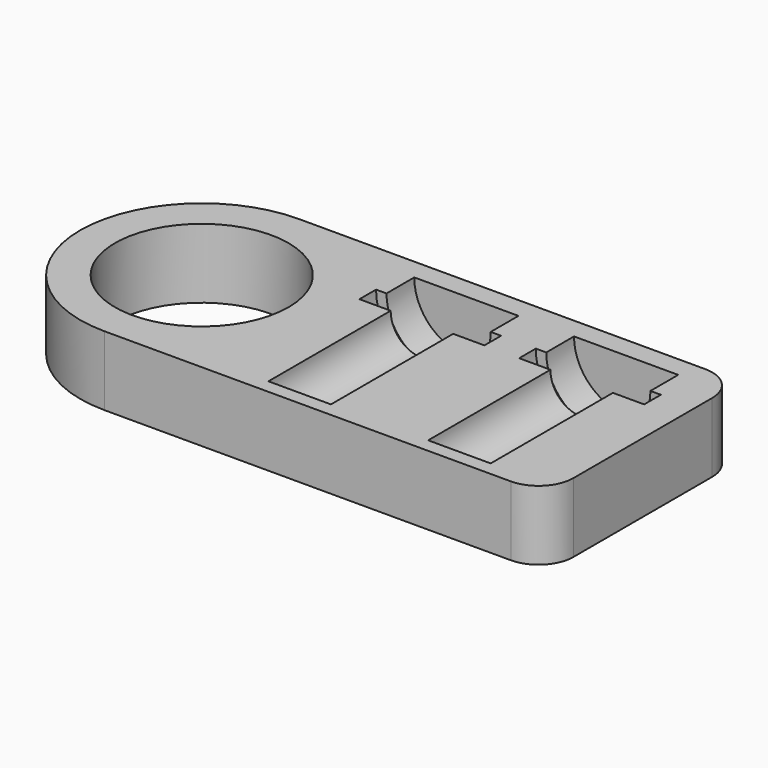
from build123d import *

# Parameters (mm, degrees)
F0_R         = 12.5
F1_DEPTH     = 10
F5_TEXT_SIZE = 5.5555555556
F6_DEPTH     = 1


# Not quite as in the source:
# - Text() gives the source's letters only with a copy of the font that has no kerning and outlines rounded to 1/6400 em; it was checked with that copy


with BuildPart() as f1:
    # F0 (on Top) → F1 (new body)
    with BuildSketch(Plane.XY):
        with BuildLine():
            ThreePointArc((0, 17.5), (5.1256313292, 5.1256313292), (17.5, 0))
            Line((17.5, 0), (76, 0))
            ThreePointArc((76, 0), (79.5355339059, 1.4644660941), (81, 5))
            Line((81, 5), (81, 30))
            ThreePointArc((81, 30), (79.5355339059, 33.5355339059), (76, 35))
            Line((76, 35), (17.5, 35))
            ThreePointArc((17.5, 35), (5.1256313292, 29.8743686708), (0, 17.5))
        make_face()
        with Locations((17.5, 17.5)):
            Circle(F0_R, mode=Mode.SUBTRACT)
    extrude(amount=F1_DEPTH)

    # F2 (on face) → F3 (revolve, cut)
    with BuildSketch(Plane.XY.offset(10)):
        Polygon((44, 24), (44, 2), (48.5, 2), (48.5, 24), (53, 24), (53, 27), (51.5, 27), (51.5, 32), (44, 32), (44, 27), align=None)
    revolve(axis=Axis((44, 13, 10), (0, 1, 0)), mode=Mode.SUBTRACT)

    # F2 (on face) → F4 (revolve, cut)
    with BuildSketch(Plane.XY.offset(10)):
        Polygon((67, 24), (67, 2), (71.5, 2), (71.5, 24), (76, 24), (76, 27), (74.5, 27), (74.5, 32), (67, 32), (67, 27), align=None)
    revolve(axis=Axis((67, 13, 10), (0, 1, 0)), mode=Mode.SUBTRACT)

    # F5 (on face) → F6 (cut)
    with BuildSketch(Plane(origin=(0, 0, 0), x_dir=(1, 0, 0), z_dir=(0, 0, -1))):
        with Locations((30, -9)):
            Text('794', F5_TEXT_SIZE, font='Open Sans', text_align=(TextAlign.LEFT, TextAlign.BOTTOM))
    extrude(amount=-F6_DEPTH, mode=Mode.SUBTRACT)


solid = f1.part
